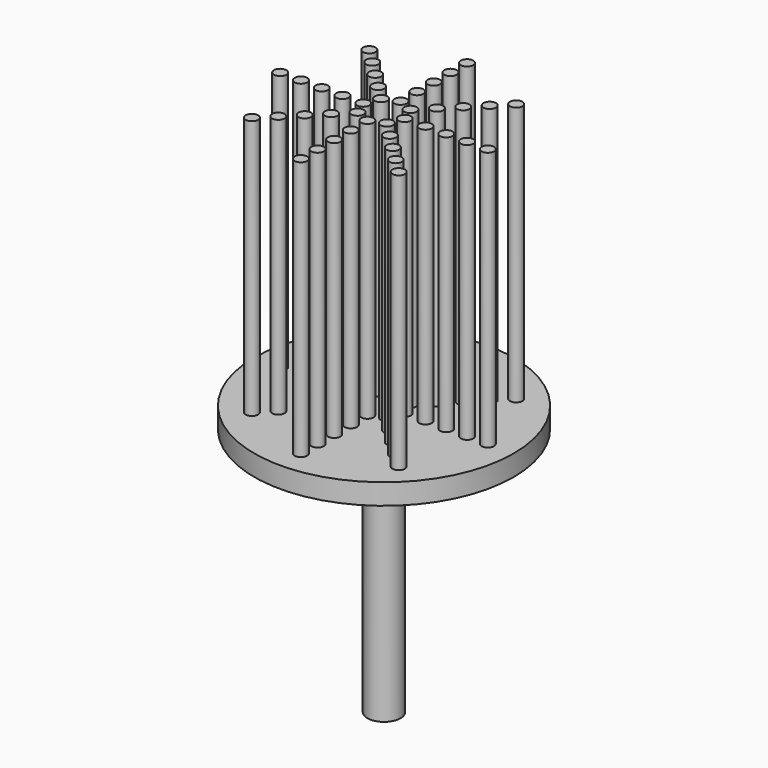
from build123d import *

# Parameters (mm, degrees)
F0_R            = 62.5
F1_DEPTH        = 10
F2_R            = 3
F3_DEPTH        = 125
F3_COPIES_COUNT = 8
F4_R            = 8
F5_DEPTH        = 120


# Not quite as in the source:
# - a pattern or mirror of a feature is missing from the dataset's text; its kind, count and spacing are read off the source's solid


with BuildPart() as f1:
    # F0 (on Top) → F1 (new body)
    with BuildSketch(Plane.XY):
        Circle(F0_R)
    extrude(amount=F1_DEPTH)

    # F2 (on face) → F3 (join)
    with BuildSketch(Plane.XY.offset(10)):
        with Locations((10, 0)):
            Circle(F2_R)
        with Locations((20, 0)):
            Circle(F2_R)
        with Locations((30, 0)):
            Circle(F2_R)
        with Locations((40, 0)):
            Circle(F2_R)
        with Locations((50, 0)):
            Circle(F2_R)
    f3 = extrude(amount=F3_DEPTH)

    # F3_copies: F3 ×8 about axis
    f3_copies_axis = Axis((0, 0, 0), (0, 0, 1))
    for i in range(1, F3_COPIES_COUNT):
        add(f3.rotate(f3_copies_axis, i * 360 / F3_COPIES_COUNT))

    # F4 (on face) → F5 (join)
    with BuildSketch(Plane.XY):
        Circle(F4_R)
    extrude(amount=-F5_DEPTH)


solid = f1.part
